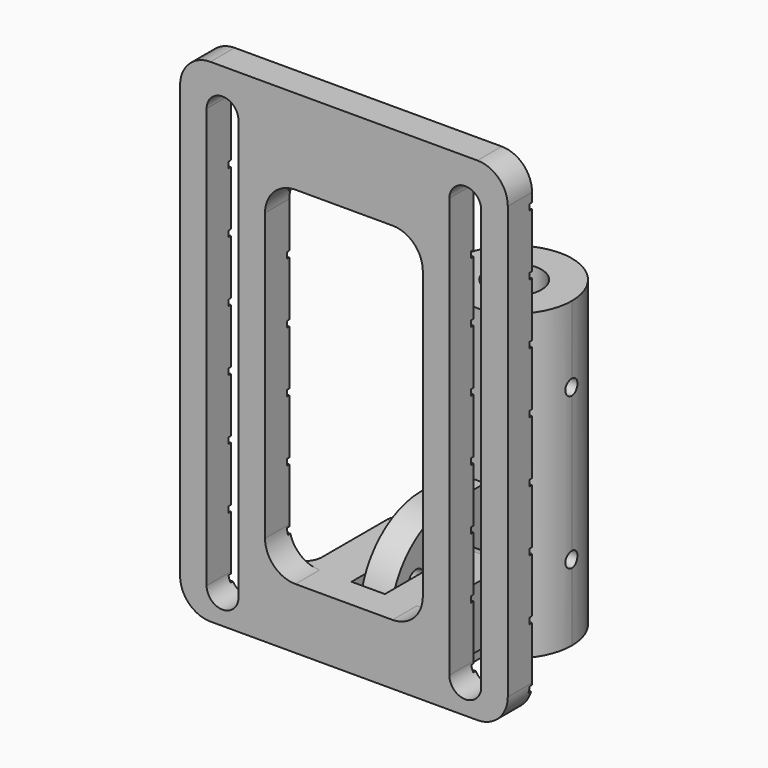
from build123d import *

# Parameters (mm, degrees)
F0_R          = 4.5
F1_DEPTH      = 50
F2_R          = 1.25
F3_DEPTH      = 12.5
F4_R          = 1.625
F4_R_2        = 2.625
F5_DEPTH      = 9.5010001262
F5_DEPTH_BACK = 9.5010001262
F7_DEPTH      = 10
F6_R          = 2.625
F6_R_2        = 1.625
F8_DEPTH      = 10
F8_DEPTH_BACK = 8
F9_DEPTH      = 2.75
F10_W         = 54
F10_H         = 81.2
F10_W_2       = 26
F10_H_2       = 57.2
F11_DEPTH     = 5
F12_T1_DEPTH  = 5
F12_T3_DEPTH  = 30
F13_R         = 2.99999
F14_W         = 54
F14_H         = 1
F15_DEPTH     = 0.5


# Not quite as in the source:
# - a fillet or chamfer that OpenCascade refuses, or shapes differently, is made with other operations: its cross-section is extruded or revolved along the edge and cut away or added
# - a fillet or chamfer is up to 0.001 mm smaller than in the source, because OpenCascade refuses the exact size
# - a feature names something its author has since deleted; it is built from what else it names


with BuildPart() as f1:
    # F0 (on Top) → F1 (new body)
    with BuildSketch(Plane.XY):
        with BuildLine():
            ThreePointArc((9.5, 0), (-5.7662812973, 7.5498344353), (-2.5, -9.1651513899))
            ThreePointArc((-2.5, -9.1651513899), (0, -9.5), (2.5, -9.1651513899))
            ThreePointArc((2.5, -9.1651513899), (7.5498344353, -5.7662812973), (9.5, 0))
        make_face()
        Circle(F0_R, mode=Mode.SUBTRACT)
        with BuildLine():
            Line((-2.5, -9.1651513899), (-2.5, -28.6651513899))
            Line((-2.5, -28.6651513899), (2.5, -28.6651513899))
            Line((2.5, -28.6651513899), (2.5, -9.1651513899))
            ThreePointArc((2.5, -9.1651513899), (0, -9.5), (-2.5, -9.1651513899))
        make_face()
    extrude(amount=F1_DEPTH)

    # F2 (on Right) → F3 (cut, symmetric)
    with BuildSketch(Plane.YZ):
        with Locations((0, 12.5)):
            Circle(F2_R)
        with Locations((0, 37.5)):
            Circle(F2_R)
    extrude(amount=F3_DEPTH, both=True, mode=Mode.SUBTRACT)

    # F4 (on Right) → F5 (cut, two sides)
    with BuildSketch(Plane.YZ) as f5_sk:
        with Locations((-16.1651513899, 20.75)):
            Circle(F4_R)
        with Locations((-20.2901513899, 19.6447095812)):
            Circle(F4_R)
        with Locations((-23.3098609711, 16.625)):
            Circle(F4_R)
        with Locations((-24.4151513899, 12.5)):
            Circle(F4_R)
        with Locations((-23.3098609711, 8.375)):
            Circle(F4_R)
        with Locations((-16.1651513899, 12.5)):
            Circle(F4_R_2)
        with Locations((-20.2901513899, 5.3552904188)):
            Circle(F4_R)
        with Locations((-16.1651513899, 4.25)):
            Circle(F4_R)
        with BuildLine():
            ThreePointArc((-16.1651513899, 0), (-25.0039861482, 3.6611652286), (-28.6651513899, 12.4999999816))
            Line((-28.6651513899, 12.4999999816), (-28.6651513899, 0))
            Line((-28.6651513899, 0), (-16.1651513899, 0))
        make_face()
        with BuildLine():
            Line((-9.1651513899, 50), (-28.6651513899, 50))
            Line((-28.6651513899, 50), (-28.6651513899, 12.4999999816))
            ThreePointArc((-28.6651513899, 12.4999999816), (-25.0039861613, 21.3388347583), (-16.1651513899, 25))
            Line((-16.1651513899, 25), (-9.1651513899, 25))
            Line((-9.1651513899, 25), (-9.1651513899, 50))
        make_face()
    extrude(amount=-F5_DEPTH, mode=Mode.SUBTRACT)
    extrude(f5_sk.sketch, amount=F5_DEPTH_BACK, mode=Mode.SUBTRACT)


with BuildPart() as f7:
    # F6 (on Right) → F7 (new body, symmetric)
    with BuildSketch(Plane.YZ):
        with BuildLine():
            ThreePointArc((-10.6651513899, 14.5), (-11.5438310464, 16.6213203436), (-13.6651513899, 17.5))
            Line((-13.6651513899, 17.5), (-30.0751513899, 17.5))
            Line((-30.0751513899, 17.5), (-30.0751513899, 7.5))
            Line((-30.0751513899, 7.5), (-13.6651513899, 7.5))
            ThreePointArc((-13.6651513899, 7.5), (-11.5438310464, 8.3786796564), (-10.6651513899, 10.5))
            Line((-10.6651513899, 10.5), (-10.6651513899, 14.5))
        make_face()
        Polygon((-27.0751513899, 10.964248284), (-27.0751513899, 14.035751716), (-24.4151513899, 15.5715034321), (-21.7551513899, 14.035751716), (-21.7551513899, 10.964248284), (-24.4151513899, 9.4284965679), align=None, mode=Mode.SUBTRACT)
        Polygon((-20.1651513899, 10.1905989232), (-20.1651513899, 14.8094010768), (-16.1651513899, 17.1188021535), (-12.1651513899, 14.8094010768), (-12.1651513899, 10.1905989232), (-16.1651513899, 7.8811978465), align=None, mode=Mode.SUBTRACT)
    extrude(amount=F7_DEPTH, both=True)

    # F6 (on Right) → F8 (join, two sides)
    with BuildSketch(Plane.YZ) as f8_sk:
        Polygon((-16.1651513899, 17.1188021535), (-20.1651513899, 14.8094010768), (-20.1651513899, 10.1905989232), (-16.1651513899, 7.8811978465), (-12.1651513899, 10.1905989232), (-12.1651513899, 14.8094010768), align=None)
        with Locations((-16.1651513899, 12.5)):
            Circle(F6_R, mode=Mode.SUBTRACT)
        Polygon((-24.4151513899, 15.5715034321), (-27.0751513899, 14.035751716), (-27.0751513899, 10.964248284), (-24.4151513899, 9.4284965679), (-21.7551513899, 10.964248284), (-21.7551513899, 14.035751716), align=None)
        with Locations((-24.4151513899, 12.5)):
            Circle(F6_R_2, mode=Mode.SUBTRACT)
    extrude(amount=F8_DEPTH)
    extrude(f8_sk.sketch, amount=-F8_DEPTH_BACK)

    # F6 (on Right) → F9 (cut, symmetric)
    with BuildSketch(Plane.YZ):
        with BuildLine():
            ThreePointArc((-10.6651513899, 14.5), (-11.5438310464, 16.6213203436), (-13.6651513899, 17.5))
            Line((-13.6651513899, 17.5), (-30.0751513899, 17.5))
            Line((-30.0751513899, 17.5), (-30.0751513899, 7.5))
            Line((-30.0751513899, 7.5), (-13.6651513899, 7.5))
            ThreePointArc((-13.6651513899, 7.5), (-11.5438310464, 8.3786796564), (-10.6651513899, 10.5))
            Line((-10.6651513899, 10.5), (-10.6651513899, 14.5))
        make_face()
        Polygon((-27.0751513899, 10.964248284), (-27.0751513899, 14.035751716), (-24.4151513899, 15.5715034321), (-21.7551513899, 14.035751716), (-21.7551513899, 10.964248284), (-24.4151513899, 9.4284965679), align=None, mode=Mode.SUBTRACT)
        Polygon((-20.1651513899, 10.1905989232), (-20.1651513899, 14.8094010768), (-16.1651513899, 17.1188021535), (-12.1651513899, 14.8094010768), (-12.1651513899, 10.1905989232), (-16.1651513899, 7.8811978465), align=None, mode=Mode.SUBTRACT)
        Polygon((-16.1651513899, 17.1188021535), (-20.1651513899, 14.8094010768), (-20.1651513899, 10.1905989232), (-16.1651513899, 7.8811978465), (-12.1651513899, 10.1905989232), (-12.1651513899, 14.8094010768), align=None)
        with Locations((-16.1651513899, 12.5)):
            Circle(F6_R, mode=Mode.SUBTRACT)
        Polygon((-24.4151513899, 15.5715034321), (-27.0751513899, 14.035751716), (-27.0751513899, 10.964248284), (-24.4151513899, 9.4284965679), (-21.7551513899, 10.964248284), (-21.7551513899, 14.035751716), align=None)
        with Locations((-24.4151513899, 12.5)):
            Circle(F6_R_2, mode=Mode.SUBTRACT)
    extrude(amount=F9_DEPTH, both=True, mode=Mode.SUBTRACT)

    # F10 (on face) → F11 (join)
    with BuildSketch(Plane.XZ.offset(30.0751513899)):
        with Locations((0, 48.1)):
            Rectangle(F10_W, F10_H)
        with BuildLine():
            ThreePointArc((-22.625, 81.7), (-20, 84.325), (-17.375, 81.7))
            Line((-17.375, 81.7), (-17.375, 12.5))
            ThreePointArc((-17.375, 12.5), (-20, 9.875), (-22.625, 12.5))
            Line((-22.625, 12.5), (-22.625, 81.7))
        make_face(mode=Mode.SUBTRACT)
        with Locations((0, 46.1)):
            Rectangle(F10_W_2, F10_H_2, mode=Mode.SUBTRACT)
        with BuildLine():
            Line((22.625, 81.7), (22.625, 12.5))
            ThreePointArc((22.625, 12.5), (20, 9.875), (17.375, 12.5))
            Line((17.375, 12.5), (17.375, 81.7))
            ThreePointArc((17.375, 81.7), (20, 84.325), (22.625, 81.7))
        make_face(mode=Mode.SUBTRACT)
    extrude(amount=F11_DEPTH)

    # F12: fillet of radius 5 on 8 edges, made by hand

    # F12_s2 → F12_t1 (join)
    with BuildSketch(Plane.XZ.offset(30.0751513899)):
        with BuildLine():
            ThreePointArc((-8, 74.7), (-11.5355339059, 73.2355339059), (-13, 69.7))
            Line((-13, 69.7), (-13, 74.7))
            Line((-13, 74.7), (-8, 74.7))
        make_face()
        with BuildLine():
            ThreePointArc((-8, 17.5), (-11.5355339059, 18.9644660941), (-13, 22.5))
            Line((-13, 22.5), (-13, 17.5))
            Line((-13, 17.5), (-8, 17.5))
        make_face()
        with BuildLine():
            ThreePointArc((8, 17.5), (11.5355339059, 18.9644660941), (13, 22.5))
            Line((13, 22.5), (13, 17.5))
            Line((13, 17.5), (8, 17.5))
        make_face()
        with BuildLine():
            ThreePointArc((13, 69.7), (11.5355339059, 73.2355339059), (8, 74.7))
            Line((8, 74.7), (13, 74.7))
            Line((13, 74.7), (13, 69.7))
        make_face()
    extrude(amount=F12_T1_DEPTH)

    # F12_s4 → F12_t3 (cut)
    with BuildSketch(Plane.XZ.offset(17.5751513899)):
        with BuildLine():
            ThreePointArc((-27, 83.7), (-25.5355339059, 87.2355339059), (-22, 88.7))
            Line((-22, 88.7), (-27, 88.7))
            Line((-27, 88.7), (-27, 83.7))
        make_face()
        with BuildLine():
            ThreePointArc((-27, 12.5), (-25.5355339059, 8.9644660941), (-22, 7.5))
            Line((-22, 7.5), (-27, 7.5))
            Line((-27, 7.5), (-27, 12.5))
        make_face()
        with BuildLine():
            ThreePointArc((22, 7.5), (25.5355339059, 8.9644660941), (27, 12.5))
            Line((27, 12.5), (27, 7.5))
            Line((27, 7.5), (22, 7.5))
        make_face()
        with BuildLine():
            ThreePointArc((22, 88.7), (25.5355339059, 87.2355339059), (27, 83.7))
            Line((27, 83.7), (27, 88.7))
            Line((27, 88.7), (22, 88.7))
        make_face()
    extrude(amount=F12_T3_DEPTH, mode=Mode.SUBTRACT)

    # F13 (radius 3 in the source; OpenCascade refuses exactly that, so slightly less here)
    f13_edges = [f7.edges().sort_by_distance(p)[0] for p in [
        (10, -30.075151, 12.5),
        (-10, -30.075151, 12.5),
    ]]
    fillet(f13_edges, radius=F13_R)

    # F14 (on face) → F15 (cut)
    with BuildSketch(Plane(origin=(0, -30.0751513899, 0), x_dir=(-1, 0, 0), z_dir=(0, 1, 0))):
        with Locations((0, 81.7)):
            Rectangle(F14_W, F14_H)
        with Locations((0, 71.7)):
            Rectangle(F14_W, F14_H)
        with Locations((0, 61.7)):
            Rectangle(F14_W, F14_H)
        with Locations((0, 51.7)):
            Rectangle(F14_W, F14_H)
        with Locations((0, 41.7)):
            Rectangle(F14_W, F14_H)
        with Locations((0, 31.7)):
            Rectangle(F14_W, F14_H)
        with Locations((0, 21.7)):
            Rectangle(F14_W, F14_H)
        with Locations((0, 11.7)):
            Rectangle(F14_W, F14_H)
    extrude(amount=-F15_DEPTH, mode=Mode.SUBTRACT)


solid = Compound([f1.part, f7.part])
